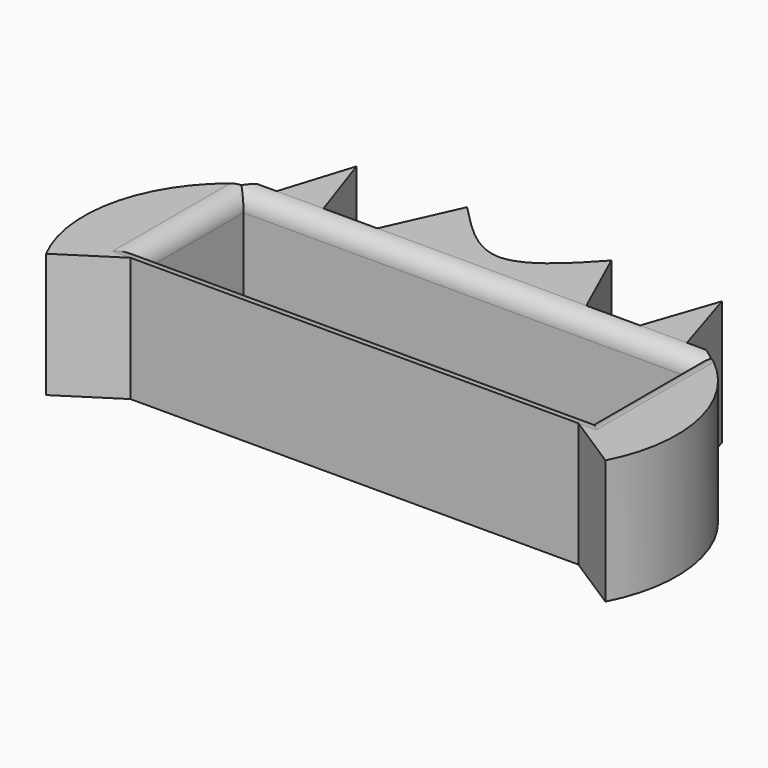
from build123d import *

# Parameters (mm, degrees)
F0_W          = 90
F0_H          = 3.590326354
F1_DEPTH      = 25
F2_T1_DEPTH   = 90
F2_T3_DEPTH   = 24.819347292
F2_T9_DEPTH   = 33.794347292
F2_S10_R      = 29.5790540859
F2_T11_DEPTH  = 19
F2_T15_DEPTH  = 98.975
F2_S16_R      = 29.5790540859
F2_T17_DEPTH  = 51
F2_T24_DEPTH  = 33.794347292
F2_S25_R      = 29.5790540859
F2_T26_DEPTH  = 19
F2_T30_DEPTH  = 98.975
F2_S31_R      = 29.5790540859
F2_T32_DEPTH  = 51
F2_T39_DEPTH  = 33.794347292
F2_S40_R      = 29.5790540859
F2_T41_DEPTH  = 19
F2_T45_DEPTH  = 98.975
F2_S46_R      = 29.5790540859
F2_T47_DEPTH  = 51
F2_T54_DEPTH  = 33.794347292
F2_S55_R      = 29.5790540859
F2_T56_DEPTH  = 19
F2_T60_DEPTH  = 98.975
F2_S61_R      = 29.5790540859
F2_T62_DEPTH  = 51
F2_T69_DEPTH  = 33.794347292
F2_T74_DEPTH  = 98.975
F2_T81_DEPTH  = 98.975
F2_T85_DEPTH  = 33.794347292
F2_T93_DEPTH  = 33.794347292
F2_T98_DEPTH  = 98.975
F2_T105_DEPTH = 98.975
F2_T109_DEPTH = 33.794347292


# Not quite as in the source:
# - a fillet or chamfer that OpenCascade refuses, or shapes differently, is made with other operations: its cross-section is extruded or revolved along the edge and cut away or added
# - a feature names something its author has since deleted; it is built from what else it names


with BuildPart() as f1:
    # F0 (on Top) → F1 (new body)
    with BuildSketch(Plane.XY):
        with BuildLine():
            Line((-56.193638593, -23.2007224411), (-45, -16))
            Line((-45, -16), (-45, -12.409673646))
            Line((-45, -12.409673646), (-45, 12.409673646))
            Line((-45, 12.409673646), (-45, 16))
            ThreePointArc((-45, 16), (-58.4287061492, -1.3639914429), (-56.193638593, -23.2007224411))
        make_face()
        with Locations((0, -14.204836823)):
            Rectangle(F0_W, F0_H)
        with BuildLine():
            Line((-21, 16), (21, 16))
            Line((21, 16), (14.5, 30.4228551942))
            add(Edge.make_bspline(
                [(-14.5, 30.4228551942), (-10.8359592966, 26.8576538948), (-0.1359775646, 13.802028979), (11.1079144259, 26.8256423781), (14.5, 30.4228551942)],
                knots=[0, 0, 0, 0, 0.5, 1, 1, 1, 1], degree=3))
            Line((-14.5, 30.4228551942), (-21, 16))
        make_face()
        with BuildLine():
            Line((45, -12.409673646), (45, -16))
            Line((45, -16), (56.193638593, -23.2007224411))
            ThreePointArc((56.193638593, -23.2007224411), (58.4287061492, -1.3639914429), (45, 16))
            Line((45, 16), (45, 12.409673646))
            Line((45, 12.409673646), (45, -12.409673646))
        make_face()
        Polygon((-36.7079592892, 30.4228551942), (-41.2157252431, 16), (-31.8110659719, 16), align=None)
        Polygon((31.8110659719, 16), (41.2157252431, 16), (36.7079592892, 30.4228551942), align=None)
        Polygon((-45, 12.409673646), (45, 12.409673646), (45, 16), (41.2157252431, 16), (31.8110659719, 16), (21, 16), (-21, 16), (-31.8110659719, 16), (-41.2157252431, 16), (-45, 16), align=None)
    extrude(amount=F1_DEPTH)

    # F2: fillet of radius 3.59 on 8 edges, made by hand

    # F2_s2 → F2_t1 (cut)
    with BuildSketch(Plane.YZ.offset(-45)):
        with BuildLine():
            ThreePointArc((12.409673646, 21.41), (13.4611603015, 23.9485133445), (15.999673646, 25))
            Line((15.999673646, 25), (12.409673646, 25))
            Line((12.409673646, 25), (12.409673646, 21.41))
        make_face()
        with BuildLine():
            ThreePointArc((12.409673646, 3.59), (13.4611603015, 1.0514866555), (15.999673646, 0))
            Line((15.999673646, 0), (12.409673646, 0))
            Line((12.409673646, 0), (12.409673646, 3.59))
        make_face()
        with BuildLine():
            ThreePointArc((-12.409673646, 3.59), (-13.4611603015, 1.0514866555), (-15.999673646, 0))
            Line((-15.999673646, 0), (-12.409673646, 0))
            Line((-12.409673646, 0), (-12.409673646, 3.59))
        make_face()
        with BuildLine():
            ThreePointArc((-12.409673646, 21.41), (-13.4611603015, 23.9485133445), (-15.999673646, 25))
            Line((-15.999673646, 25), (-12.409673646, 25))
            Line((-12.409673646, 25), (-12.409673646, 21.41))
        make_face()
    extrude(amount=F2_T1_DEPTH, mode=Mode.SUBTRACT)

    # F2_s4 → F2_t3 (cut)
    with BuildSketch(Plane.XZ.offset(-12.409673646)):
        with BuildLine():
            ThreePointArc((-45, 21.41), (-46.0514866555, 23.9485133445), (-48.59, 25))
            Line((-48.59, 25), (-45, 25))
            Line((-45, 25), (-45, 21.41))
        make_face()
        with BuildLine():
            ThreePointArc((-45, 3.59), (-46.0514866555, 1.0514866555), (-48.59, 0))
            Line((-48.59, 0), (-45, 0))
            Line((-45, 0), (-45, 3.59))
        make_face()
        with BuildLine():
            ThreePointArc((45, 21.41), (46.0514866555, 23.9485133445), (48.59, 25))
            Line((48.59, 25), (45, 25))
            Line((45, 25), (45, 21.41))
        make_face()
        with BuildLine():
            ThreePointArc((45, 3.59), (46.0514866555, 1.0514866555), (48.59, 0))
            Line((48.59, 0), (45, 0))
            Line((45, 0), (45, 3.59))
        make_face()
    extrude(amount=F2_T3_DEPTH, mode=Mode.SUBTRACT)


with BuildPart() as f2_tool7:
    # F2_s8 → F2_t9 (new body)
    with BuildSketch(Plane.XZ.offset(12.409673646)):
        with BuildLine():
            ThreePointArc((-45, 21.41), (-46.0514866555, 23.9485133445), (-48.59, 25))
            Line((-48.59, 25), (-45, 25))
            Line((-45, 25), (-45, 21.41))
        make_face()
    extrude(amount=-F2_T9_DEPTH)

    # F2_s10 → F2_t11 (intersect, symmetric)
    with BuildSketch(Plane.XY.offset(23.2)):
        with Locations((-29.9864788785, -9.4855767867)):
            Circle(F2_S10_R)
    extrude(amount=F2_T11_DEPTH, both=True, mode=Mode.INTERSECT)

    split(bisect_by=Plane.XZ.offset(-12.409673646), keep=Keep.BOTTOM)


with BuildPart() as f2_tool13:
    # F2_s14 → F2_t15 (new body)
    with BuildSketch(Plane.YZ.offset(-53.975)):
        with BuildLine():
            ThreePointArc((12.409673646, 21.41), (13.4611603015, 23.9485133445), (15.999673646, 25))
            Line((15.999673646, 25), (12.409673646, 25))
            Line((12.409673646, 25), (12.409673646, 21.41))
        make_face()
    extrude(amount=F2_T15_DEPTH)

    # F2_s16 → F2_t17 (intersect, symmetric)
    with BuildSketch(Plane.XY.offset(23.2)):
        with Locations((-29.9864788785, -9.4855767867)):
            Circle(F2_S16_R)
    extrude(amount=F2_T17_DEPTH, both=True, mode=Mode.INTERSECT)

    split(bisect_by=Plane.YZ.offset(-45), keep=Keep.BOTTOM)


with BuildPart() as f2_tool7_1:
    add(f2_tool7.part)

    # F2_t19: intersect F2_tool13
    add(f2_tool13.part, mode=Mode.INTERSECT)


with BuildPart() as f1_1:
    add(f1.part)

    # F2_t5: cut F2_tool7
    add(f2_tool7_1.part, mode=Mode.SUBTRACT)


with BuildPart() as f2_tool22:
    # F2_s23 → F2_t24 (new body)
    with BuildSketch(Plane.XZ.offset(-21.384673646)):
        with BuildLine():
            ThreePointArc((45, 21.41), (46.0514866555, 23.9485133445), (48.59, 25))
            Line((48.59, 25), (45, 25))
            Line((45, 25), (45, 21.41))
        make_face()
    extrude(amount=F2_T24_DEPTH)

    # F2_s25 → F2_t26 (intersect, symmetric)
    with BuildSketch(Plane.XY.offset(23.2)):
        with Locations((29.9864788785, -9.4855767867)):
            Circle(F2_S25_R)
    extrude(amount=F2_T26_DEPTH, both=True, mode=Mode.INTERSECT)

    split(bisect_by=Plane.XZ.offset(-12.409673646), keep=Keep.BOTTOM)


with BuildPart() as f2_tool28:
    # F2_s29 → F2_t30 (new body)
    with BuildSketch(Plane.YZ.offset(-45)):
        with BuildLine():
            ThreePointArc((12.409673646, 21.41), (13.4611603015, 23.9485133445), (15.999673646, 25))
            Line((15.999673646, 25), (12.409673646, 25))
            Line((12.409673646, 25), (12.409673646, 21.41))
        make_face()
    extrude(amount=F2_T30_DEPTH)

    # F2_s31 → F2_t32 (intersect, symmetric)
    with BuildSketch(Plane.XY.offset(23.2)):
        with Locations((29.9864788785, -9.4855767867)):
            Circle(F2_S31_R)
    extrude(amount=F2_T32_DEPTH, both=True, mode=Mode.INTERSECT)

    split(bisect_by=Plane.YZ.offset(45), keep=Keep.TOP)


with BuildPart() as f2_tool22_1:
    add(f2_tool22.part)

    # F2_t34: intersect F2_tool28
    add(f2_tool28.part, mode=Mode.INTERSECT)


with BuildPart() as f1_2:
    add(f1_1.part)

    # F2_t20: cut F2_tool22
    add(f2_tool22_1.part, mode=Mode.SUBTRACT)


with BuildPart() as f2_tool37:
    # F2_s38 → F2_t39 (new body)
    with BuildSketch(Plane.XZ.offset(12.409673646)):
        with BuildLine():
            ThreePointArc((-45, 3.59), (-46.0514866555, 1.0514866555), (-48.59, 0))
            Line((-48.59, 0), (-45, 0))
            Line((-45, 0), (-45, 3.59))
        make_face()
    extrude(amount=-F2_T39_DEPTH)

    # F2_s40 → F2_t41 (intersect, symmetric)
    with BuildSketch(Plane.XY.offset(1.8)):
        with Locations((-29.9864788785, -9.4855767867)):
            Circle(F2_S40_R)
    extrude(amount=F2_T41_DEPTH, both=True, mode=Mode.INTERSECT)

    split(bisect_by=Plane.XZ.offset(-12.409673646), keep=Keep.BOTTOM)


with BuildPart() as f2_tool43:
    # F2_s44 → F2_t45 (new body)
    with BuildSketch(Plane.YZ.offset(-53.975)):
        with BuildLine():
            ThreePointArc((12.409673646, 3.59), (13.4611603015, 1.0514866555), (15.999673646, 0))
            Line((15.999673646, 0), (12.409673646, 0))
            Line((12.409673646, 0), (12.409673646, 3.59))
        make_face()
    extrude(amount=F2_T45_DEPTH)

    # F2_s46 → F2_t47 (intersect, symmetric)
    with BuildSketch(Plane.XY.offset(1.8)):
        with Locations((-29.9864788785, -9.4855767867)):
            Circle(F2_S46_R)
    extrude(amount=F2_T47_DEPTH, both=True, mode=Mode.INTERSECT)

    split(bisect_by=Plane.YZ.offset(-45), keep=Keep.BOTTOM)


with BuildPart() as f2_tool37_1:
    add(f2_tool37.part)

    # F2_t49: intersect F2_tool43
    add(f2_tool43.part, mode=Mode.INTERSECT)


with BuildPart() as f1_3:
    add(f1_2.part)

    # F2_t35: cut F2_tool37
    add(f2_tool37_1.part, mode=Mode.SUBTRACT)


with BuildPart() as f2_tool52:
    # F2_s53 → F2_t54 (new body)
    with BuildSketch(Plane.XZ.offset(-21.384673646)):
        with BuildLine():
            ThreePointArc((45, 3.59), (46.0514866555, 1.0514866555), (48.59, 0))
            Line((48.59, 0), (45, 0))
            Line((45, 0), (45, 3.59))
        make_face()
    extrude(amount=F2_T54_DEPTH)

    # F2_s55 → F2_t56 (intersect, symmetric)
    with BuildSketch(Plane.XY.offset(1.8)):
        with Locations((29.9864788785, -9.4855767867)):
            Circle(F2_S55_R)
    extrude(amount=F2_T56_DEPTH, both=True, mode=Mode.INTERSECT)

    split(bisect_by=Plane.XZ.offset(-12.409673646), keep=Keep.BOTTOM)


with BuildPart() as f2_tool58:
    # F2_s59 → F2_t60 (new body)
    with BuildSketch(Plane.YZ.offset(-45)):
        with BuildLine():
            ThreePointArc((12.409673646, 3.59), (13.4611603015, 1.0514866555), (15.999673646, 0))
            Line((15.999673646, 0), (12.409673646, 0))
            Line((12.409673646, 0), (12.409673646, 3.59))
        make_face()
    extrude(amount=F2_T60_DEPTH)

    # F2_s61 → F2_t62 (intersect, symmetric)
    with BuildSketch(Plane.XY.offset(1.8)):
        with Locations((29.9864788785, -9.4855767867)):
            Circle(F2_S61_R)
    extrude(amount=F2_T62_DEPTH, both=True, mode=Mode.INTERSECT)

    split(bisect_by=Plane.YZ.offset(45), keep=Keep.TOP)


with BuildPart() as f2_tool52_1:
    add(f2_tool52.part)

    # F2_t64: intersect F2_tool58
    add(f2_tool58.part, mode=Mode.INTERSECT)


with BuildPart() as f1_4:
    add(f1_3.part)

    # F2_t50: cut F2_tool52
    add(f2_tool52_1.part, mode=Mode.SUBTRACT)


with BuildPart() as f2_tool67:
    # F2_s68 → F2_t69 (new body)
    with BuildSketch(Plane.XZ.offset(-12.409673646)):
        with BuildLine():
            ThreePointArc((45, 3.59), (46.0514866555, 1.0514866555), (48.59, 0))
            Line((48.59, 0), (45, 0))
            Line((45, 0), (45, 3.59))
        make_face()
    extrude(amount=F2_T69_DEPTH)

    split(bisect_by=Plane.XZ.offset(16), keep=Keep.BOTTOM)

    split(bisect_by=Plane.XZ.offset(12.409673646), keep=Keep.TOP)


with BuildPart() as f2_tool72:
    # F2_s73 → F2_t74 (new body)
    with BuildSketch(Plane.YZ.offset(53.975)):
        with BuildLine():
            ThreePointArc((-12.409673646, 3.59), (-13.4611603015, 1.0514866555), (-15.999673646, 0))
            Line((-15.999673646, 0), (-12.409673646, 0))
            Line((-12.409673646, 0), (-12.409673646, 3.59))
        make_face()
    extrude(amount=-F2_T74_DEPTH)

    split(bisect_by=Plane.YZ.offset(45), keep=Keep.TOP)


with BuildPart() as f2_tool67_1:
    add(f2_tool67.part)

    # F2_t76: intersect F2_tool72
    add(f2_tool72.part, mode=Mode.INTERSECT)


with BuildPart() as f1_5:
    add(f1_4.part)

    # F2_t65: cut F2_tool67
    add(f2_tool67_1.part, mode=Mode.SUBTRACT)


with BuildPart() as f2_tool79:
    # F2_s80 → F2_t81 (new body)
    with BuildSketch(Plane.YZ.offset(45)):
        with BuildLine():
            ThreePointArc((-12.409673646, 3.59), (-13.4611603015, 1.0514866555), (-15.999673646, 0))
            Line((-15.999673646, 0), (-12.409673646, 0))
            Line((-12.409673646, 0), (-12.409673646, 3.59))
        make_face()
    extrude(amount=-F2_T81_DEPTH)

    split(bisect_by=Plane.YZ.offset(-45), keep=Keep.BOTTOM)


with BuildPart() as f2_tool83:
    # F2_s84 → F2_t85 (new body)
    with BuildSketch(Plane.XZ.offset(21.384673646)):
        with BuildLine():
            ThreePointArc((-45, 3.59), (-46.0514866555, 1.0514866555), (-48.59, 0))
            Line((-48.59, 0), (-45, 0))
            Line((-45, 0), (-45, 3.59))
        make_face()
    extrude(amount=-F2_T85_DEPTH)

    split(bisect_by=Plane.XZ.offset(16), keep=Keep.BOTTOM)

    split(bisect_by=Plane.XZ.offset(12.409673646), keep=Keep.TOP)


with BuildPart() as f2_tool79_1:
    add(f2_tool79.part)

    # F2_t88: intersect F2_tool83
    add(f2_tool83.part, mode=Mode.INTERSECT)


with BuildPart() as f1_6:
    add(f1_5.part)

    # F2_t77: cut F2_tool79
    add(f2_tool79_1.part, mode=Mode.SUBTRACT)


with BuildPart() as f2_tool91:
    # F2_s92 → F2_t93 (new body)
    with BuildSketch(Plane.XZ.offset(-12.409673646)):
        with BuildLine():
            ThreePointArc((45, 21.41), (46.0514866555, 23.9485133445), (48.59, 25))
            Line((48.59, 25), (45, 25))
            Line((45, 25), (45, 21.41))
        make_face()
    extrude(amount=F2_T93_DEPTH)

    split(bisect_by=Plane.XZ.offset(16), keep=Keep.BOTTOM)

    split(bisect_by=Plane.XZ.offset(12.409673646), keep=Keep.TOP)


with BuildPart() as f2_tool96:
    # F2_s97 → F2_t98 (new body)
    with BuildSketch(Plane.YZ.offset(53.975)):
        with BuildLine():
            ThreePointArc((-12.409673646, 21.41), (-13.4611603015, 23.9485133445), (-15.999673646, 25))
            Line((-15.999673646, 25), (-12.409673646, 25))
            Line((-12.409673646, 25), (-12.409673646, 21.41))
        make_face()
    extrude(amount=-F2_T98_DEPTH)

    split(bisect_by=Plane.YZ.offset(45), keep=Keep.TOP)


with BuildPart() as f2_tool91_1:
    add(f2_tool91.part)

    # F2_t100: intersect F2_tool96
    add(f2_tool96.part, mode=Mode.INTERSECT)


with BuildPart() as f1_7:
    add(f1_6.part)

    # F2_t89: cut F2_tool91
    add(f2_tool91_1.part, mode=Mode.SUBTRACT)


with BuildPart() as f2_tool103:
    # F2_s104 → F2_t105 (new body)
    with BuildSketch(Plane.YZ.offset(45)):
        with BuildLine():
            ThreePointArc((-12.409673646, 21.41), (-13.4611603015, 23.9485133445), (-15.999673646, 25))
            Line((-15.999673646, 25), (-12.409673646, 25))
            Line((-12.409673646, 25), (-12.409673646, 21.41))
        make_face()
    extrude(amount=-F2_T105_DEPTH)

    split(bisect_by=Plane.YZ.offset(-45), keep=Keep.BOTTOM)


with BuildPart() as f2_tool107:
    # F2_s108 → F2_t109 (new body)
    with BuildSketch(Plane.XZ.offset(21.384673646)):
        with BuildLine():
            ThreePointArc((-45, 21.41), (-46.0514866555, 23.9485133445), (-48.59, 25))
            Line((-48.59, 25), (-45, 25))
            Line((-45, 25), (-45, 21.41))
        make_face()
    extrude(amount=-F2_T109_DEPTH)

    split(bisect_by=Plane.XZ.offset(16), keep=Keep.BOTTOM)

    split(bisect_by=Plane.XZ.offset(12.409673646), keep=Keep.TOP)


with BuildPart() as f2_tool103_1:
    add(f2_tool103.part)

    # F2_t112: intersect F2_tool107
    add(f2_tool107.part, mode=Mode.INTERSECT)


with BuildPart() as f1_8:
    add(f1_7.part)

    # F2_t101: cut F2_tool103
    add(f2_tool103_1.part, mode=Mode.SUBTRACT)


solid = f1_8.part
